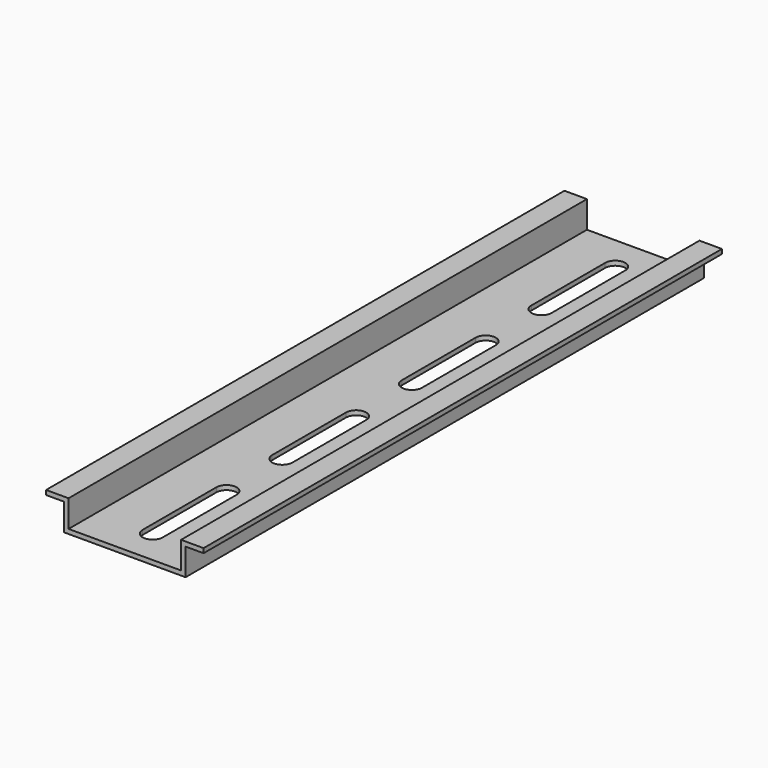
from build123d import *

# Parameters (mm, degrees)
F1_DEPTH = 144
F3_DEPTH = 1.001


# Not quite as in the source:
# - a feature names something its author has since deleted; it is built from what else it names


with BuildPart() as f1:
    # F0 (on Front) → F1 (new body)
    with BuildSketch(Plane.XZ):
        Polygon((-17.5, 6), (-17.5, 5), (-13.5, 5), (-13.5, -1), (13.5, -1), (13.5, 5), (17.5, 5), (17.5, 6), (12.5, 6), (12.5, 0), (-12.5, 0), (-12.5, 6), align=None)
    extrude(amount=F1_DEPTH)

    # F2 (on face) → F3 (cut, through all)
    with BuildSketch(Plane.XY):
        with BuildLine():
            ThreePointArc((-2.25, -28.25), (0, -30.5), (2.25, -28.25))
            Line((2.25, -28.25), (2.25, -7.75))
            ThreePointArc((2.25, -7.75), (0, -5.5), (-2.25, -7.75))
            Line((-2.25, -7.75), (-2.25, -28.25))
        make_face()
        with BuildLine():
            Line((-2.25, -43.75), (-2.25, -64.25))
            ThreePointArc((-2.25, -64.25), (0, -66.5), (2.25, -64.25))
            Line((2.25, -64.25), (2.25, -43.75))
            ThreePointArc((2.25, -43.75), (0, -41.5), (-2.25, -43.75))
        make_face()
        with BuildLine():
            Line((-2.25, -79.75), (-2.25, -100.25))
            ThreePointArc((-2.25, -100.25), (0, -102.5), (2.25, -100.25))
            Line((2.25, -100.25), (2.25, -79.75))
            ThreePointArc((2.25, -79.75), (0, -77.5), (-2.25, -79.75))
        make_face()
        with BuildLine():
            Line((-2.25, -115.75), (-2.25, -136.25))
            ThreePointArc((-2.25, -136.25), (0, -138.5), (2.25, -136.25))
            Line((2.25, -136.25), (2.25, -115.75))
            ThreePointArc((2.25, -115.75), (0, -113.5), (-2.25, -115.75))
        make_face()
    extrude(amount=-F3_DEPTH, mode=Mode.SUBTRACT)


solid = f1.part
